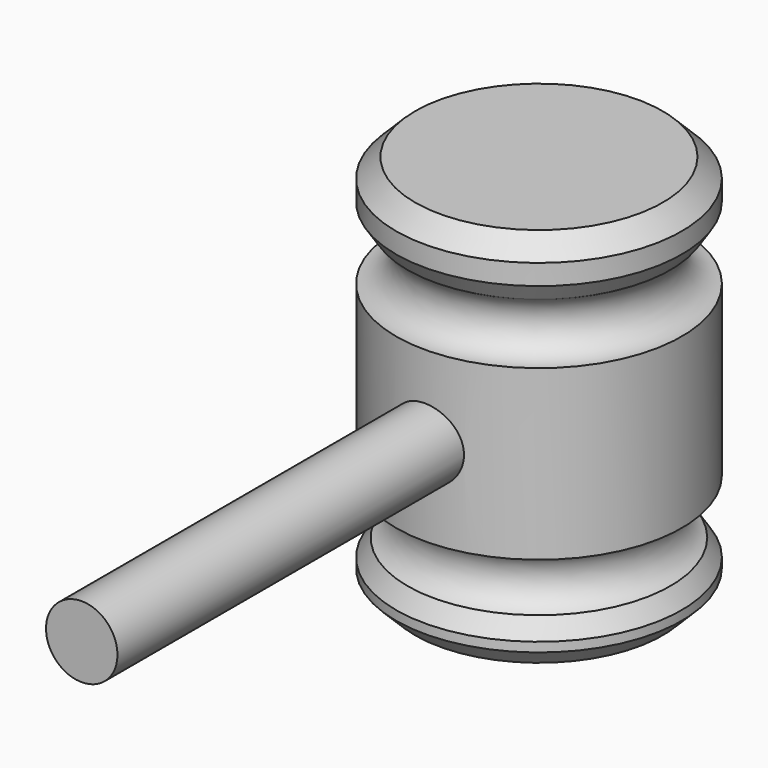
from build123d import *

# Parameters (mm, degrees)
F2_R     = 9.525
F3_DEPTH = 152.4


# Not quite as in the source:
# - a fillet or chamfer that OpenCascade refuses, or shapes differently, is made with other operations: its cross-section is extruded or revolved along the edge and cut away or added


with BuildPart() as f1:
    # F0 (on Front) → F1 (revolve)
    with BuildSketch(Plane.XZ):
        with BuildLine():
            Line((-38.1, 0), (0, 0))
            Line((0, 0), (0, 101.6))
            Line((0, 101.6), (-38.1, 101.6))
            Line((-38.1, 101.6), (-38.1, 87.0632982802))
            ThreePointArc((-38.1, 87.0632982802), (-30.48, 79.4432982802), (-38.1, 71.8232982802))
            Line((-38.1, 71.8232982802), (-38.1, 26.8419931632))
            ThreePointArc((-38.1, 26.8419931632), (-30.48, 19.2219931632), (-38.1, 11.6019931632))
            Line((-38.1, 11.6019931632), (-38.1, 0))
        make_face()
    revolve(axis=Axis((0, 0, 50.8), (0, 0, 1)))

    # F2 (on Front) → F3 (join)
    with BuildSketch(Plane.XZ):
        with Locations((0, 49.7302636504)):
            Circle(F2_R)
    extrude(amount=F3_DEPTH)

    # F4: chamfer of 5.08 on 6 edges, made by hand

    # F4_s1 → F4_t2 (revolve, cut)
    with BuildSketch(Plane.XZ):
        Polygon((-38.1, 96.52), (-33.02, 101.6), (-38.1, 101.6), align=None)
    revolve(axis=Axis((0, 0, 101.6), (0, 0, 1)), mode=Mode.SUBTRACT)

    # F4_s3 → F4_t4 (revolve, cut)
    with BuildSketch(Plane.XZ):
        with BuildLine():
            Line((-35.052, 86.4271436394), (-38.1, 91.0830405454))
            Line((-38.1, 91.0830405454), (-38.1, 87.0632982802))
            ThreePointArc((-38.1, 87.0632982802), (-36.4706968515, 86.8870722727), (-35.052, 86.4271436394))
        make_face()
    revolve(axis=Axis((0, 0, 87.0632982802), (0, 0, 1)), mode=Mode.SUBTRACT)

    # F4_s5 → F4_t6 (revolve, cut)
    with BuildSketch(Plane.XZ):
        with BuildLine():
            Line((-38.1, 7.582250898), (-35.052, 12.2381478041))
            ThreePointArc((-35.052, 12.2381478041), (-36.4706968515, 11.7782191708), (-38.1, 11.6019931632))
            Line((-38.1, 11.6019931632), (-38.1, 7.582250898))
        make_face()
    revolve(axis=Axis((0, 0, 11.6019931632), (0, 0, 1)), mode=Mode.SUBTRACT)

    # F4_s7 → F4_t8 (revolve, cut)
    with BuildSketch(Plane.XZ):
        Polygon((-33.02, 0), (-38.1, 5.08), (-38.1, 0), align=None)
    revolve(axis=Axis((0, 0, 0), (0, 0, 1)), mode=Mode.SUBTRACT)


solid = f1.part
